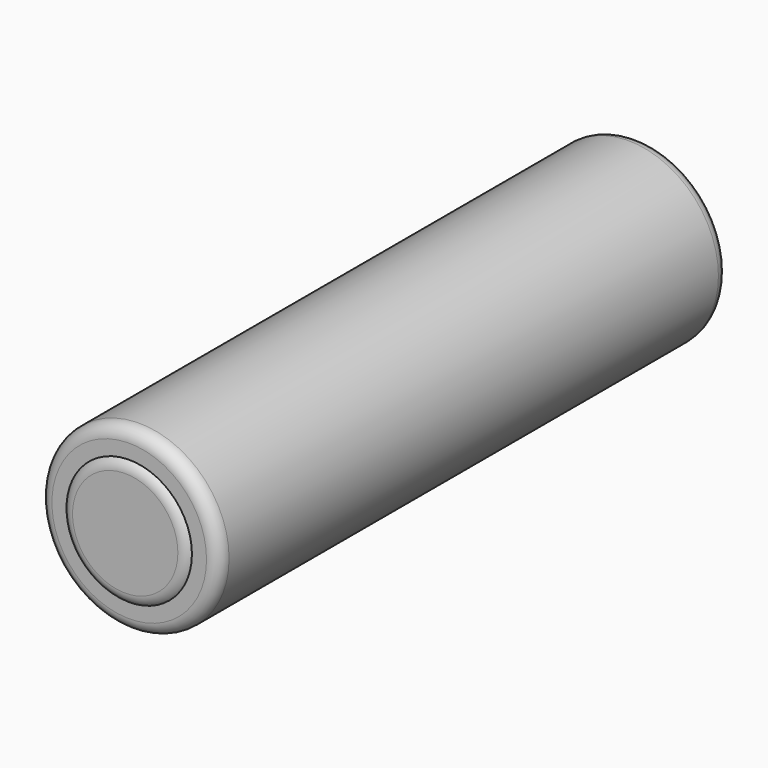
from build123d import *

# Parameters (mm, degrees)
F0_R     = 9.09955
F1_DEPTH = 64.4906
F2_R     = 6.35
F3_DEPTH = 0.508


# Not quite as in the source:
# - a fillet or chamfer that OpenCascade refuses, or shapes differently, is made with other operations: its cross-section is extruded or revolved along the edge and cut away or added


with BuildPart() as f1:
    # F0 (on Front) → F1 (new body)
    with BuildSketch(Plane.XZ):
        Circle(F0_R)
    extrude(amount=-F1_DEPTH)

    # F2 (on face) → F3 (join)
    with BuildSketch(Plane.XZ):
        Circle(F2_R)
    extrude(amount=F3_DEPTH)

    # F4: fillet of radius 1.27 on 3 edges, made by hand

    # F4_s1 → F4_t2 (revolve, cut)
    with BuildSketch(Plane.XY):
        with BuildLine():
            ThreePointArc((9.09955, 63.2206), (8.7275756121, 64.1186256121), (7.82955, 64.4906))
            Line((7.82955, 64.4906), (9.09955, 64.4906))
            Line((9.09955, 64.4906), (9.09955, 63.2206))
        make_face()
    revolve(axis=Axis((0, 64.4906, 0), (0, -1, 0)), mode=Mode.SUBTRACT)

    # F4_s3 → F4_t4 (revolve, cut)
    with BuildSketch(Plane.XY):
        with BuildLine():
            ThreePointArc((9.09955, 1.27), (8.7275756121, 0.3719743879), (7.82955, 0))
            Line((7.82955, 0), (9.09955, 0))
            Line((9.09955, 0), (9.09955, 1.27))
        make_face()
    revolve(axis=Axis((0, 0, 0), (0, -1, 0)), mode=Mode.SUBTRACT)

    # F4_s5 → F4_t6 (revolve, cut)
    with BuildSketch(Plane.XY):
        with BuildLine():
            ThreePointArc((6.35, 0), (5.9019612663, -0.3739225326), (5.334, -0.508))
            Line((5.334, -0.508), (6.35, -0.508))
            Line((6.35, -0.508), (6.35, 0))
        make_face()
    revolve(axis=Axis((0, -0.508, 0), (0, -1, 0)), mode=Mode.SUBTRACT)


solid = f1.part
